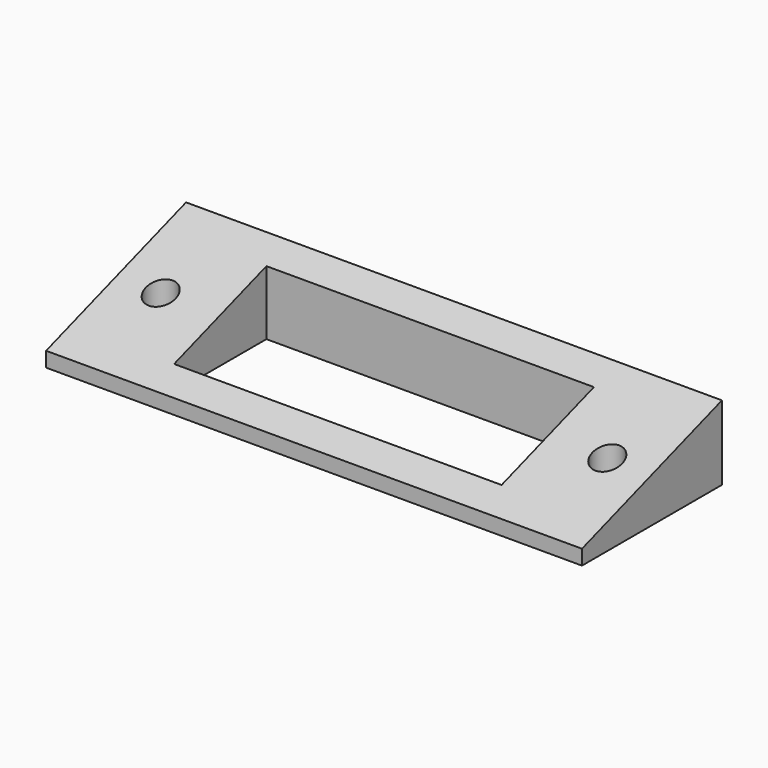
from build123d import *

# Parameters (mm, degrees)
F0_W        = 72
F0_H        = 23.5
F0_R        = 2
F0_W_2      = 44
F0_H_2      = 15.5
F1_DEPTH    = 2
F2_DEPTH    = 8
F3_T1_DEPTH = 193.9586602962


# Not quite as in the source:
# - a fillet or chamfer that OpenCascade refuses, or shapes differently, is made with other operations: its cross-section is extruded or revolved along the edge and cut away or added


with BuildPart() as f1:
    # F0 (on Top) → F1 (new body)
    with BuildSketch(Plane.XY):
        with Locations((36, -11.75)):
            Rectangle(F0_W, F0_H)
        with Locations((6, -11.75)):
            Circle(F0_R, mode=Mode.SUBTRACT)
        with Locations((36, -11.75)):
            Rectangle(F0_W_2, F0_H_2, mode=Mode.SUBTRACT)
        with Locations((66, -11.75)):
            Circle(F0_R, mode=Mode.SUBTRACT)
    extrude(amount=F1_DEPTH)

    # F2 (add): a face of the model
    f2_faces = [f1.faces().sort_by_distance(p)[0] for p in [
        (36, -0.7573803536, 2),
    ]]
    extrude(f2_faces, amount=F2_DEPTH)

    # F3: chamfer of 23.5 x 8 on 1 edges, made by hand

    # F3_s2 → F3_t1 (cut)
    with BuildSketch(Plane.YZ.offset(-60.9793301481)):
        Polygon((-23.5, 2), (0, 10), (-23.5, 10), align=None)
    extrude(amount=F3_T1_DEPTH, mode=Mode.SUBTRACT)


solid = f1.part
